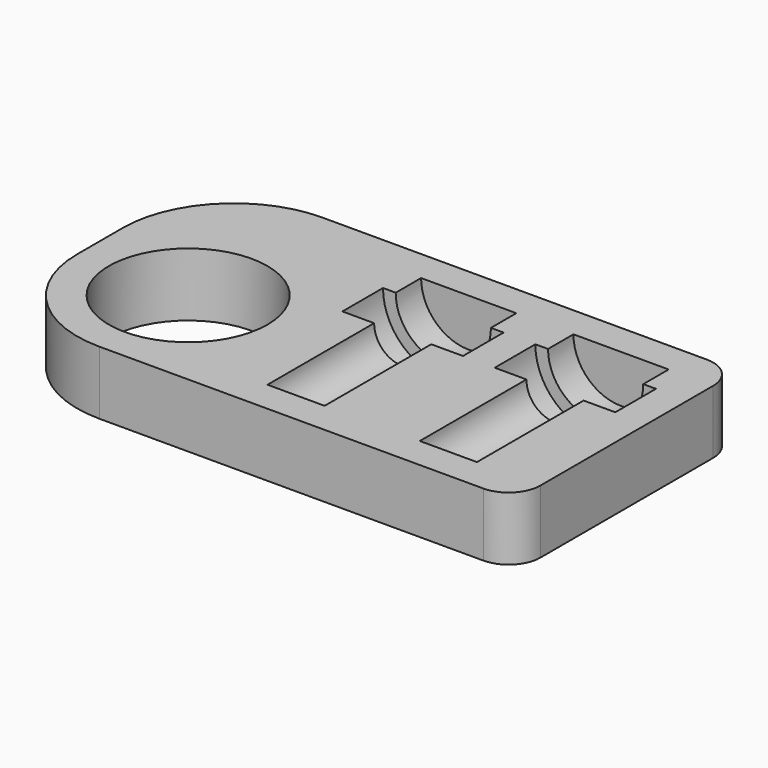
from build123d import *

# Parameters (mm, degrees)
F0_R         = 12.5
F1_DEPTH     = 10
F5_TEXT_SIZE = 5.5555555556
F6_DEPTH     = 1


# Not quite as in the source:
# - Text() gives the source's letters only with a copy of the font that has no kerning and outlines rounded to 1/6400 em; it was checked with that copy


with BuildPart() as f1:
    # F0 (on Top) → F1 (new body)
    with BuildSketch(Plane.XY):
        with BuildLine():
            ThreePointArc((0, 17.5), (5.1256313292, 5.1256313292), (17.5, 0))
            Line((17.5, 0), (78, 0))
            ThreePointArc((78, 0), (81.5355339059, 1.4644660941), (83, 5))
            Line((83, 5), (83, 39))
            ThreePointArc((83, 39), (81.5355339059, 42.5355339059), (78, 44))
            Line((78, 44), (17.5, 44))
            ThreePointArc((17.5, 44), (5.1256313292, 38.8743686708), (0, 26.5))
            Line((0, 26.5), (0, 17.5))
        make_face()
        with Locations((17.5, 17.5)):
            Circle(F0_R, mode=Mode.SUBTRACT)
    extrude(amount=F1_DEPTH)

    # F2 (on face) → F3 (revolve, cut)
    with BuildSketch(Plane.XY.offset(10)):
        Polygon((44.5, 26), (44.5, 5), (49, 5), (49, 26), (54, 26), (54, 34), (52, 34), (52, 39), (44.5, 39), (44.5, 34), align=None)
    revolve(axis=Axis((44.5, 15.5, 10), (0, 1, 0)), mode=Mode.SUBTRACT)

    # F2 (on face) → F4 (revolve, cut)
    with BuildSketch(Plane.XY.offset(10)):
        Polygon((68.5, 26), (68.5, 5), (73, 5), (73, 26), (78, 26), (78, 34), (76, 34), (76, 39), (68.5, 39), (68.5, 34), align=None)
    revolve(axis=Axis((68.5, 15.5, 10), (0, 1, 0)), mode=Mode.SUBTRACT)

    # F5 (on face) → F6 (cut)
    with BuildSketch(Plane(origin=(0, 0, 0), x_dir=(1, 0, 0), z_dir=(0, 0, -1))):
        with Locations((30, -9)):
            Text('818', F5_TEXT_SIZE, font='Open Sans', text_align=(TextAlign.LEFT, TextAlign.BOTTOM))
    extrude(amount=-F6_DEPTH, mode=Mode.SUBTRACT)


solid = f1.part
